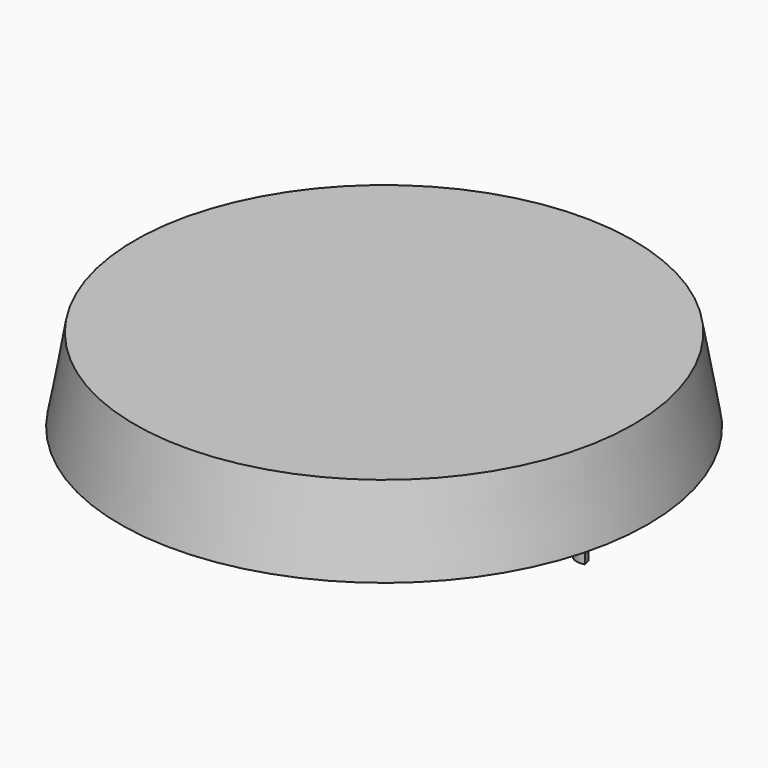
from build123d import *

# Parameters (mm, degrees)
F0_R           = 30
F1_DEPTH       = 10
F1_TAPER       = -10
F2_TEXT_SIZE   = 11.687751104
F2_TEXT_SIZE_2 = 7.250755287
F2_TEXT_SIZE_3 = 10.5332455563
F3_DEPTH       = 2


# Not quite as in the source:
# - Text() gives the source's letters only with a copy of the font that has no kerning and outlines rounded to 1/6400 em; it was checked with that copy


with BuildPart() as f1:
    # F0 (on Top) → F1 (new body)
    with BuildSketch(Plane.XY):
        Circle(F0_R)
    extrude(amount=-F1_DEPTH, taper=F1_TAPER)

    # F2 (on face) → F3 (join)
    with BuildSketch(Plane(origin=(0, 0, -10), x_dir=(1, 0, 0), z_dir=(0, 0, -1))):
        with Locations((-25, -9.4151807949)):
            Text('Johansson', F2_TEXT_SIZE, font='Open Sans', font_style=FontStyle.ITALIC, text_align=(TextAlign.LEFT, TextAlign.BOTTOM))
        with Locations((-22, 11.4160631995)):
            Text('fam.', F2_TEXT_SIZE_2, font='Open Sans', font_style=FontStyle.ITALIC, text_align=(TextAlign.LEFT, TextAlign.BOTTOM))
        with Locations((-29.5, 1.4160631995)):
            Text('Witthammar', F2_TEXT_SIZE_3, font='Open Sans', font_style=FontStyle.ITALIC, text_align=(TextAlign.LEFT, TextAlign.BOTTOM))
    extrude(amount=F3_DEPTH)


solid = f1.part
